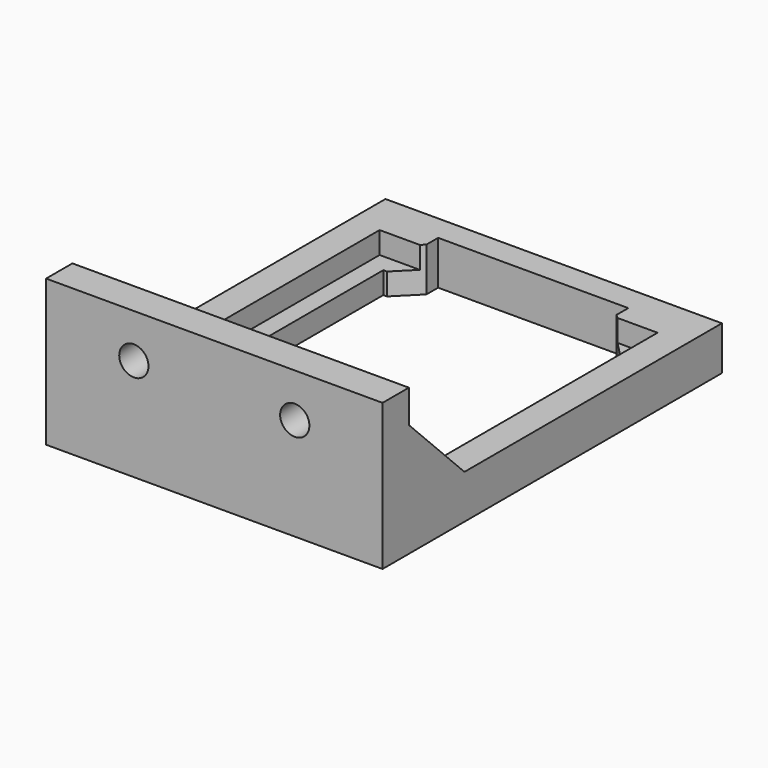
from build123d import *

# Parameters (mm, degrees)
F0_W          = 46
F0_H          = 58
F1_DEPTH      = 6
F2_W          = 38
F2_H          = 38
F3_DEPTH      = 3
F4_W          = 33
F4_H          = 33
F5_DEPTH      = 3.001
F6_W          = 26
F6_H          = 5
F7_DEPTH      = 3.001
F7_DEPTH_BACK = 3.001
F8_W          = 26
F8_H          = 5
F9_DEPTH      = 3.001
F9_DEPTH_BACK = 3.001
F10_SIZE      = 3
F11_W         = 4.5
F11_H         = 20
F12_DEPTH     = 46
F13_W         = 4
F13_H         = 9.5
F14_DEPTH     = 10
F15_T4_DEPTH  = 4
F16_W         = 4
F16_H         = 9.5
F17_DEPTH     = 10
F18_T4_DEPTH  = 4
F19_R         = 2
F20_DEPTH     = 4.501


# Not quite as in the source:
# - a fillet or chamfer that OpenCascade refuses, or shapes differently, is made with other operations: its cross-section is extruded or revolved along the edge and cut away or added


with BuildPart() as f1:
    # F0 (on Top) → F1 (new body)
    with BuildSketch(Plane.XY):
        Rectangle(F0_W, F0_H)
    extrude(amount=F1_DEPTH)

    # F2 (on face) → F3 (cut)
    with BuildSketch(Plane.XY.offset(6)):
        with Locations((0, 4)):
            Rectangle(F2_W, F2_H)
    extrude(amount=-F3_DEPTH, mode=Mode.SUBTRACT)

    # F4 (on face) → F5 (cut, through all)
    with BuildSketch(Plane.XY.offset(3)):
        with Locations((0, 4)):
            Rectangle(F4_W, F4_H)
    extrude(amount=-F5_DEPTH, mode=Mode.SUBTRACT)

    # F6 (on face) → F7 (cut, two sides)
    with BuildSketch(Plane.XY.offset(3)) as f7_sk:
        with Locations((0, 23)):
            Rectangle(F6_W, F6_H)
    extrude(amount=-F7_DEPTH, mode=Mode.SUBTRACT)
    extrude(f7_sk.sketch, amount=F7_DEPTH_BACK, mode=Mode.SUBTRACT)

    # F8 (on face) → F9 (cut, two sides)
    with BuildSketch(Plane.XY.offset(3)) as f9_sk:
        with Locations((0, -15)):
            Rectangle(F8_W, F8_H)
    extrude(amount=F9_DEPTH, mode=Mode.SUBTRACT)
    extrude(f9_sk.sketch, amount=-F9_DEPTH_BACK, mode=Mode.SUBTRACT)

    # F10
    f10_edges = [f1.edges().sort_by_distance(p)[0] for p in [
        (-13, -12.5, 1.5),
        (-13, 20.5, 1.5),
        (13, 20.5, 1.5),
        (13, -12.5, 1.5),
    ]]
    chamfer(f10_edges, length=F10_SIZE)

    # F11 (on face) → F12 (join)
    with BuildSketch(Plane(origin=(-23, 0, 0), x_dir=(0, -1, 0), z_dir=(-1, 0, 0))):
        with Locations((26.75, 10)):
            Rectangle(F11_W, F11_H)
    extrude(amount=-F12_DEPTH)

    # F13 (on face) → F14 (join)
    with BuildSketch(Plane.XY.offset(6)):
        with Locations((-21, -19.75)):
            Rectangle(F13_W, F13_H)
    extrude(amount=F14_DEPTH)

    # F15: chamfer of 10 on 1 edges, made by hand


with BuildPart() as f15_tool2:
    # F15_s3 → F15_t4 (new body)
    with BuildSketch(Plane.YZ.offset(-19)):
        with BuildLine():
            Line((-14.7171572875, 5.7171572875), (-25.2828427125, 16.2828427125))
            Line((-25.2828427125, 16.2828427125), (-25.2828427125, 16.4828427125))
            ThreePointArc((-25.2828427125, 16.4828427125), (-20.1414213562, 16.2), (-15, 16.2))
            Line((-15, 16.2), (-14.8, 16))
            ThreePointArc((-14.8, 16), (-14.8, 10.8585786438), (-14.5171572875, 5.7171572875))
            Line((-14.5171572875, 5.7171572875), (-14.7171572875, 5.7171572875))
        make_face()
    extrude(amount=-F15_T4_DEPTH)

    split(bisect_by=Plane.XY.offset(6), keep=Keep.TOP)

    split(bisect_by=Plane.XZ.offset(24.5), keep=Keep.BOTTOM)


with BuildPart() as f1_1:
    add(f1.part)

    # F15_t1: cut F15_tool2
    add(f15_tool2.part, mode=Mode.SUBTRACT)

    # F16 (on face) → F17 (join)
    with BuildSketch(Plane.XY.offset(6)):
        with Locations((21, -19.75)):
            Rectangle(F16_W, F16_H)
    extrude(amount=F17_DEPTH)

    # F18: chamfer of 10 on 1 edges, made by hand


with BuildPart() as f18_tool2:
    # F18_s3 → F18_t4 (new body)
    with BuildSketch(Plane.YZ.offset(23)):
        with BuildLine():
            Line((-14.7171572875, 5.7171572875), (-25.2828427125, 16.2828427125))
            Line((-25.2828427125, 16.2828427125), (-25.2828427125, 16.4828427125))
            ThreePointArc((-25.2828427125, 16.4828427125), (-20.1414213562, 16.2), (-15, 16.2))
            Line((-15, 16.2), (-14.8, 16))
            ThreePointArc((-14.8, 16), (-14.8, 10.8585786438), (-14.5171572875, 5.7171572875))
            Line((-14.5171572875, 5.7171572875), (-14.7171572875, 5.7171572875))
        make_face()
    extrude(amount=-F18_T4_DEPTH)

    split(bisect_by=Plane.XY.offset(6), keep=Keep.TOP)

    split(bisect_by=Plane.XZ.offset(24.5), keep=Keep.BOTTOM)


with BuildPart() as f1_2:
    add(f1_1.part)

    # F18_t1: cut F18_tool2
    add(f18_tool2.part, mode=Mode.SUBTRACT)

    # F19 (on face) → F20 (cut, through all)
    with BuildSketch(Plane(origin=(0, -24.5, 0), x_dir=(-1, 0, 0), z_dir=(0, 1, 0))):
        with Locations((11, 14)):
            Circle(F19_R)
        with Locations((-11, 14)):
            Circle(F19_R)
    extrude(amount=-F20_DEPTH, mode=Mode.SUBTRACT)


solid = f1_2.part
